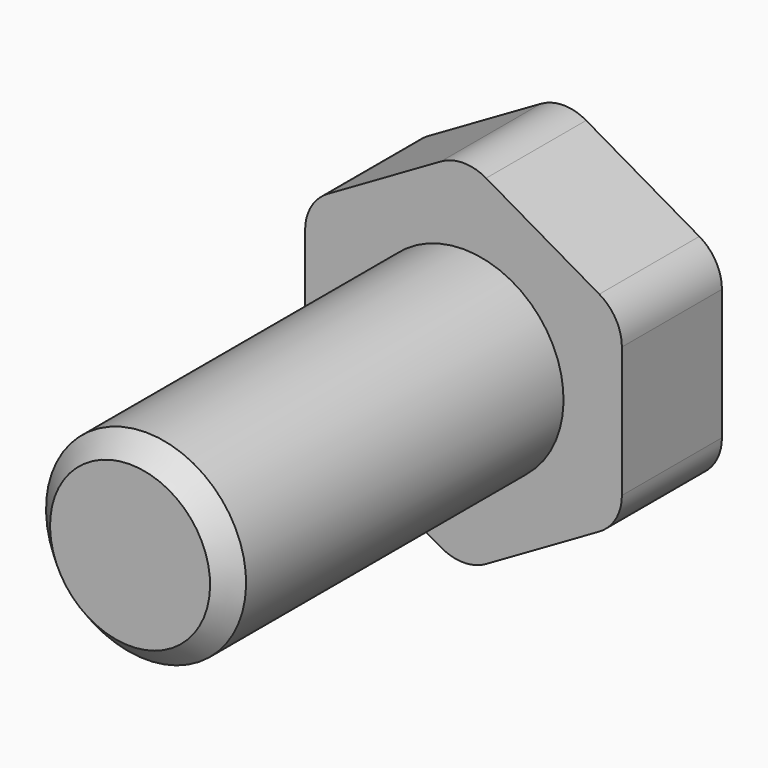
from build123d import *

# Parameters (mm, degrees)
F2_R     = 15.825
F3_DEPTH = 25


# Not quite as in the source:
# - a feature names something its author has since deleted; it is built from what else it names


with BuildPart() as f1:
    # F0 (on Right) → F1 (revolve)
    with BuildSketch(Plane.YZ):
        Polygon((0, 15.825), (0, 6), (-23.8, 6), (-25, 4.8), (-25, 0), (7.5, 0), (7.5, 15.825), align=None)
    revolve(axis=Axis((0, -8.75, 0), (0, -1, 0)))

    # F2 (on face) → F3 (cut)
    with BuildSketch(Plane(origin=(0, 7.5, 0), x_dir=(-1, 0, 0), z_dir=(0, 1, 0))):
        Circle(F2_R)
        with BuildLine():
            ThreePointArc((1.3563466521, -10.1865680099), (0, -10.55), (-1.3563466521, -10.1865680099))
            Line((-1.3563466521, -10.1865680099), (-8.1436533479, -6.267914662))
            ThreePointArc((-8.1436533479, -6.267914662), (-9.1365680099, -5.275), (-9.5, -3.9186533479))
            Line((-9.5, -3.9186533479), (-9.5, 3.9186533479))
            ThreePointArc((-9.5, 3.9186533479), (-9.1365680099, 5.275), (-8.1436533479, 6.267914662))
            Line((-8.1436533479, 6.267914662), (-1.3563466521, 10.1865680099))
            ThreePointArc((-1.3563466521, 10.1865680099), (0, 10.55), (1.3563466521, 10.1865680099))
            Line((1.3563466521, 10.1865680099), (8.1436533479, 6.267914662))
            ThreePointArc((8.1436533479, 6.267914662), (9.1365680099, 5.275), (9.5, 3.9186533479))
            Line((9.5, 3.9186533479), (9.5, -3.9186533479))
            ThreePointArc((9.5, -3.9186533479), (9.1365680099, -5.275), (8.1436533479, -6.267914662))
            Line((8.1436533479, -6.267914662), (1.3563466521, -10.1865680099))
        make_face(mode=Mode.SUBTRACT)
    extrude(amount=-F3_DEPTH, mode=Mode.SUBTRACT)


solid = f1.part
